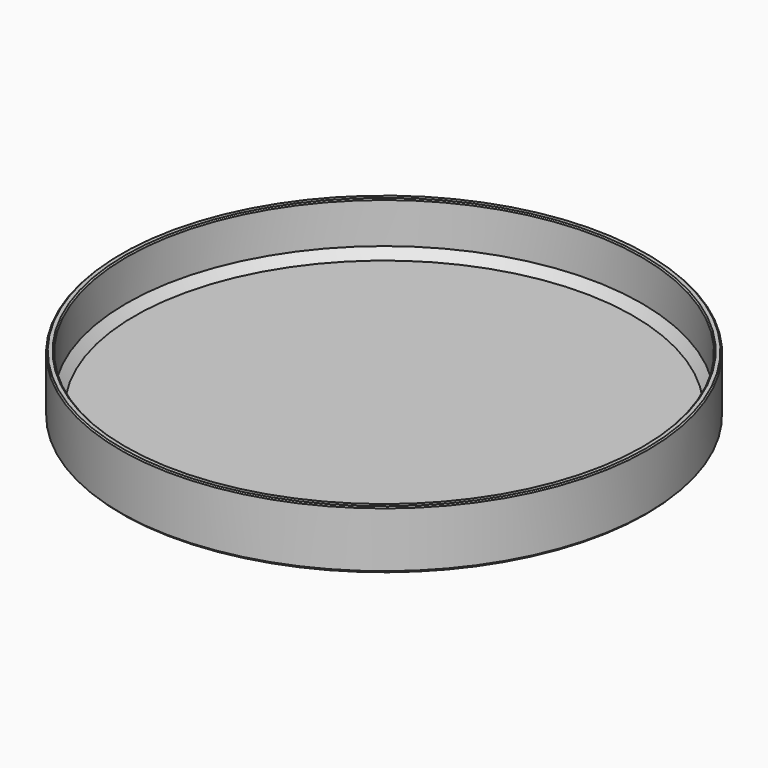
from build123d import *

# Parameters (mm, degrees)
F0_R     = 63.1
F0_R_2   = 61.6
F1_DEPTH = 2
F2_DEPTH = 14
F3_SIZE  = 0.5
F4_SIZE  = 2
F5_SIZE  = 0.3


# Not quite as in the source:
# - a feature names something its author has since deleted; it is built from what else it names


with BuildPart() as f1:
    # F0 (on Top) → F1 (new body)
    with BuildSketch(Plane.XY):
        Circle(F0_R)
        Circle(F0_R_2, mode=Mode.SUBTRACT)
        Circle(F0_R_2)
    extrude(amount=F1_DEPTH)

    # F0 (on Top) → F2 (join)
    with BuildSketch(Plane.XY):
        Circle(F0_R)
        Circle(F0_R_2, mode=Mode.SUBTRACT)
    extrude(amount=F2_DEPTH)

    # F3
    f3_edges = [f1.edges().sort_by_distance(p)[0] for p in [
        (-63.1, 0, 0),
    ]]
    chamfer(f3_edges, length=F3_SIZE)

    # F4
    f4_edges = [f1.edges().sort_by_distance(p)[0] for p in [
        (-61.6, 0, 2),
    ]]
    chamfer(f4_edges, length=F4_SIZE)

    # F5
    f5_edges = [f1.edges().sort_by_distance(p)[0] for p in [
        (-63.1, 0, 14),
        (-61.6, 0, 14),
    ]]
    chamfer(f5_edges, length=F5_SIZE)


solid = f1.part
